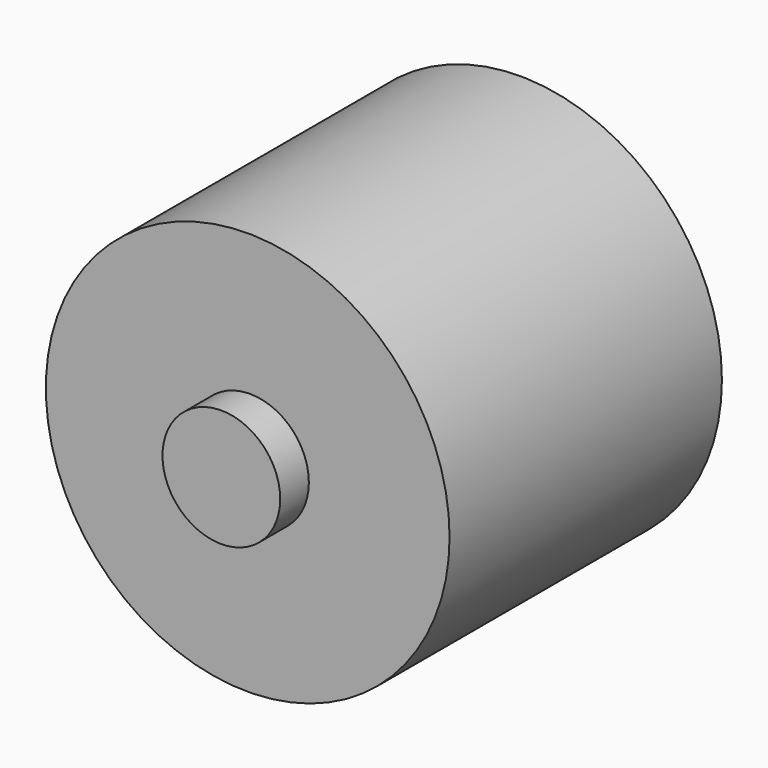
from build123d import *

# Parameters (mm, degrees)
F4_R     = 17.1690350151
F5_DEPTH = 28.956
F6_R     = 5.0050524863
F7_DEPTH = 32.004


# Not quite as in the source:
# - a feature of the source that left no trace in its solid (it failed there, or was rolled back) is left out
# - the program builds the solid bodies; features that only make, move or delete a surface that nothing else refers to are left out


with BuildPart() as f5:
    # F4 (on Front) → F5 (new body)
    with BuildSketch(Plane.XZ):
        with Locations((2.4482863955, 4.896572791)):
            Circle(F4_R)
    extrude(amount=F5_DEPTH)

    # F6 (on Front) → F7 (join)
    with BuildSketch(Plane.XZ):
        with Locations((2.6441500522, 5.0924359821)):
            Circle(F6_R)
    extrude(amount=F7_DEPTH)


solid = f5.part
